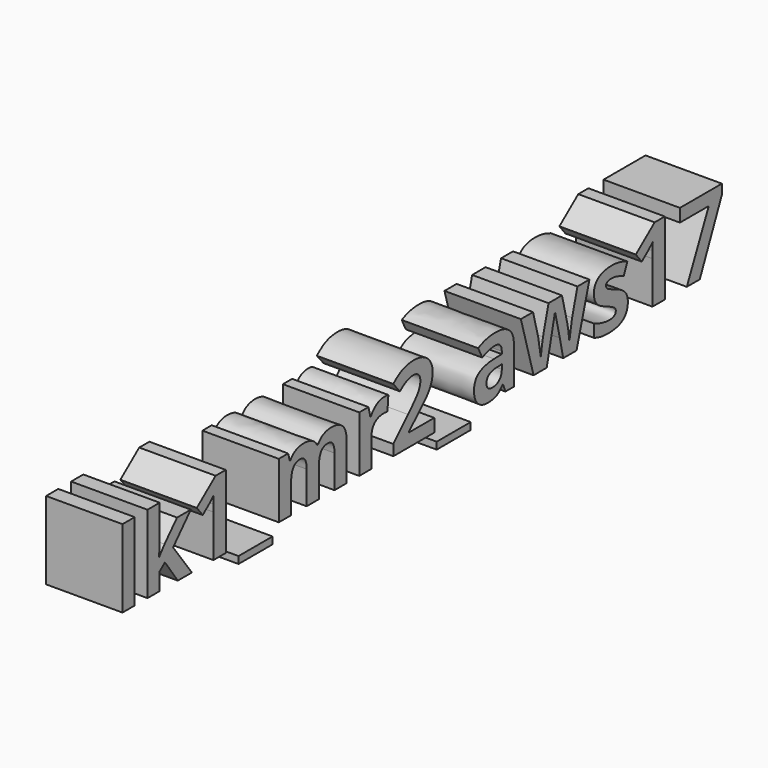
from build123d import *

# Parameters (mm, degrees)
F0_TEXT_SIZE = 34.0632399472
F1_DEPTH     = 25.4


# Not quite as in the source:
# - Text() gives the source's letters only with a copy of the font that has no kerning and outlines rounded to 1/6400 em; it was checked with that copy


with BuildPart() as f1:
    # F0 (on Right) → F1 (new body)
    with BuildSketch(Plane.YZ):
        with Locations((-127, 0)):
            Text('lk1_mr2_aws17', F0_TEXT_SIZE, font='Open Sans', font_style=FontStyle.BOLD, text_align=(TextAlign.LEFT, TextAlign.BOTTOM))
    extrude(amount=F1_DEPTH)


solid = f1.part
